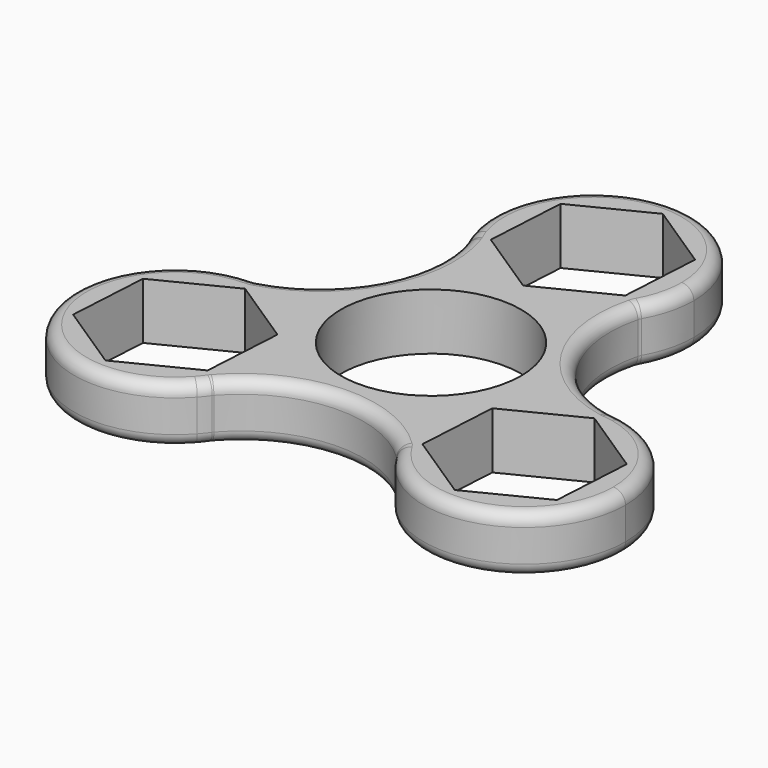
from build123d import *

# Parameters (mm, degrees)
F0_R     = 11.15
F1_DEPTH = 7
F2_F1_R  = 1.5
F2_F2_R  = 1.5


with BuildPart() as f1:
    # F0 (on Top) → F1 (new body)
    with BuildSketch(Plane.XY):
        with BuildLine():
            ThreePointArc((10.8701441505, 18.7190770861), (12.1321748255, 21.7475059655), (12.5627389416, 25))
            ThreePointArc((12.5627389416, 25), (-1.9408257651, 37.338384354), (-11.7949776129, 21.0446797713))
            ThreePointArc((-11.7949776129, 21.0446797713), (-11.4827733825, 20.3271653092), (-11.2080382122, 19.5944859312))
            ThreePointArc((-11.2080382122, 19.5944859312), (-0.4325019607, 12.5098143949), (10.8701441505, 18.7190770861))
        make_face()
        Polygon((9.089622183, 29.5385804257), (8.5067065081, 19.4517800088), (-0.5201767333, 14.9131995832), (-8.9641442997, 20.4614195743), (-8.3812286248, 30.5482199912), (0.6456546165, 35.0868004168), align=None, mode=Mode.SUBTRACT)
        with BuildLine():
            ThreePointArc((-11.2080382122, 19.5944859312), (-11.4827733825, 20.3271653092), (-11.7949776129, 21.0446797713))
            ThreePointArc((-11.7949776129, 21.0446797713), (-11.5242179862, 20.3103913648), (-11.2080382122, 19.5944859312))
        make_face()
        with BuildLine():
            ThreePointArc((22.6181682998, -0.1217200611), (12.635395047, 6.7366942627), (10.8701441505, 18.7190770861))
            ThreePointArc((10.8701441505, 18.7190770861), (-0.4325019607, 12.5098143949), (-11.2080382122, 19.5944859312))
            ThreePointArc((-11.2080382122, 19.5944859312), (-12.1562126199, 7.5199435321), (-21.6506350946, 0))
            ThreePointArc((-21.6506350946, 0), (-12.8349108913, -3.6737578493), (-9.1863712928, -12.4999489169))
            ThreePointArc((-9.1863712928, -12.4999489169), (-9.7446636362, -16.1939465134), (-11.3696702118, -19.5579712181))
            ThreePointArc((-11.3696702118, -19.5579712181), (-0.4387225513, -14.3418431428), (10.8209508199, -18.8042824341))
            ThreePointArc((10.8209508199, -18.8042824341), (11.0948946462, -5.9112724262), (22.6181682998, -0.1217200611))
        make_face()
        Circle(F0_R, mode=Mode.SUBTRACT)
        with BuildLine():
            ThreePointArc((24.1675427061, -0.3385125497), (23.3900548392, -0.2501321134), (22.6181682998, -0.1217200611))
            ThreePointArc((22.6181682998, -0.1217200611), (11.0948946462, -5.9112724262), (10.8209508199, -18.8042824341))
            ThreePointArc((10.8209508199, -18.8042824341), (24.8820677095, -24.6639415332), (34.164092227, -12.5852564312))
            ThreePointArc((34.164092227, -12.5852564312), (31.3476641659, -4.68092632), (24.1675427061, -0.3385125497))
        make_face()
        Polygon((30.6909754684, -8.0466760055), (30.1080597935, -18.1334764223), (21.0811765521, -22.672056848), (12.6372089857, -17.1238368569), (13.2201246606, -7.03703644), (22.2470079019, -2.4984560143), align=None, mode=Mode.SUBTRACT)
        with BuildLine():
            ThreePointArc((24.1675427061, -0.3385125497), (23.3962504791, -0.2058530615), (22.6181682998, -0.1217200611))
            ThreePointArc((22.6181682998, -0.1217200611), (23.3900548392, -0.2501321134), (24.1675427061, -0.3385125497))
        make_face()
        with BuildLine():
            ThreePointArc((-9.1863712928, -12.4999489169), (-12.8349108913, -3.6737578493), (-21.6506350946, 0))
            ThreePointArc((-21.6506350946, 0), (-33.0930942669, -17.6123525583), (-12.3321052174, -20.7913725696))
            ThreePointArc((-12.3321052174, -20.7913725696), (-11.8668215808, -20.1622385439), (-11.3696702118, -19.5579712181))
            ThreePointArc((-11.3696702118, -19.5579712181), (-9.7446636362, -16.1939465134), (-9.1863712928, -12.4999489169))
        make_face()
        Polygon((-22.2692869677, -22.5867493337), (-30.7132545342, -17.0385293426), (-30.1303388592, -6.9517289257), (-21.1034556179, -2.4131485), (-12.6594880515, -7.9613684912), (-13.2424037264, -18.048168908), align=None, mode=Mode.SUBTRACT)
        with BuildLine():
            ThreePointArc((-11.3696702118, -19.5579712181), (-11.8668215808, -20.1622385439), (-12.3321052174, -20.7913725696))
            ThreePointArc((-12.3321052174, -20.7913725696), (-11.831572617, -20.1897436513), (-11.3696702118, -19.5579712181))
        make_face()
    extrude(amount=F1_DEPTH)

    # F2: fillet of radius 1.5 on 12 edges, made by hand

    # F2_f1
    f2_f1_edges = [f1.edges().sort_by_distance(p)[0] for p in [
        (10.8209508199, -18.8042824341, 3.5),
        (22.6181682998, -0.1217200611, 3.5),
        (10.8701441505, 18.7190770861, 3.5),
        (-11.2080382122, 19.5944859312, 3.5),
        (-21.6506350946, 0, 3.5),
        (-11.3696702118, -19.5579712181, 3.5),
    ]]
    fillet(f2_f1_edges, radius=F2_F1_R)

    # F2_f2
    f2_f2_edges = [f1.edges().sort_by_distance(p)[0] for p in [
        (32.2611908869, -19.2148491783, 0),
        (32.2611908869, -19.2148491783, 7),
        (0.5055853475, 37.4921530194, 0),
        (0.5055853475, 37.4921530194, 7),
        (-32.7263163585, -18.3625091891, 0),
        (-32.7263163585, -18.3625091891, 7),
        (-21.6417928421, 0.0141676529, 7),
        (-11.3648950422, -19.5558017338, 7),
        (-21.6417928421, 0.0141676529, 0),
        (-11.3648950422, -19.5558017338, 0),
        (10.8779925716, 18.7043356443, 7),
        (-11.2085469685, 19.5892657708, 7),
        (10.8779925716, 18.7043356443, 0),
        (-11.2085469685, 19.5892657708, 0),
        (10.8042601464, -18.8037086452, 7),
        (22.6139018865, -0.1186693851, 7),
        (10.8042601464, -18.8037086452, 0),
        (22.6139018865, -0.1186693851, 0),
    ]]
    fillet(f2_f2_edges, radius=F2_F2_R)


solid = f1.part
